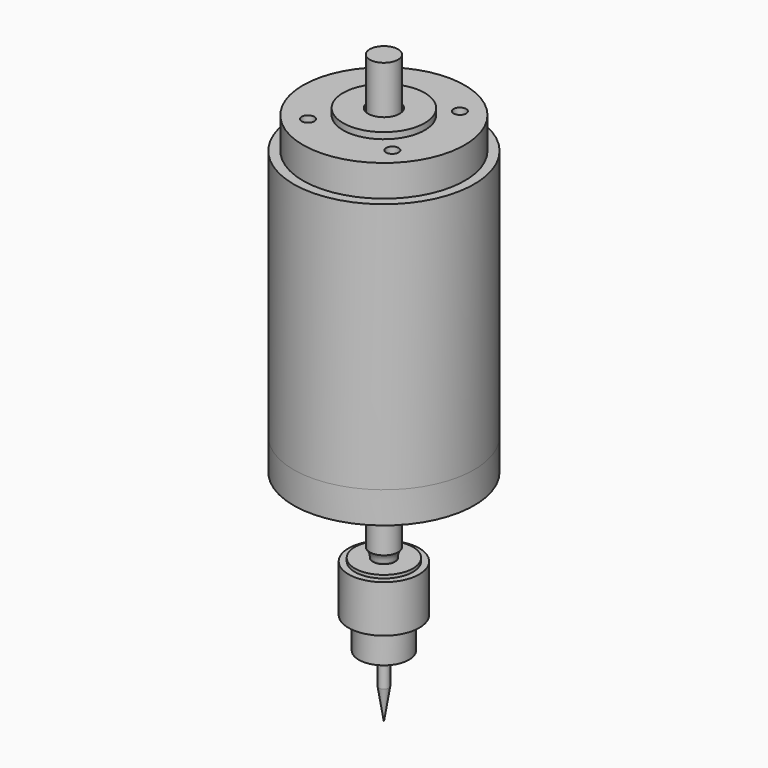
from build123d import *

# Parameters (mm, degrees)
F0_W      = 3
F0_H      = 80
F4_OFFSET = 0.5
F6_R      = 2
F7_DEPTH  = 10


# Not quite as in the source:
# - a fillet or chamfer that OpenCascade refuses, or shapes differently, is made with other operations: its cross-section is extruded or revolved along the edge and cut away or added


with BuildPart() as f1:
    # F0 (on Front) → F1 (revolve)
    with BuildSketch(Plane.XZ):
        Polygon((0, 100), (0, 102), (-13, 102), (-13, 100), (-25.75, 100), (-25.75, 90), (-25.75, 10), (-28.75, 10), (-28.75, 0), (-25.75, 0), (0, 0), align=None)
    revolve(axis=Axis((0, 0, 33.5), (0, 0, 1)))


with BuildPart() as f2:
    # F0 (on Front) → F2 (revolve)
    with BuildSketch(Plane.XZ):
        Polygon((4.5, 117), (0, 117), (0, 102), (0, 100), (0, 0), (0, -50), (1.5875, -50), (8, -50), (8, -41), (11.25, -40), (11.25, -25), (9.25, -25), (9.25, -24), (3.5, -24), (3.5, -21), (4.5, -21), align=None)
        Polygon((1.5875, -50), (0, -50), (0, -70), (1.5875, -60), align=None)
    revolve(axis=Axis((0, 0, 33.5), (0, 0, 1)))


with BuildPart() as f3:
    # F0 (on Front) → F3 (revolve)
    with BuildSketch(Plane.XZ):
        with Locations((-27.25, 50)):
            Rectangle(F0_W, F0_H)
    revolve(axis=Axis((0, 0, 33.5), (0, 0, 1)))


with BuildPart() as f1_1:
    add(f1.part)

    # F4: cut F2, made larger all round first
    f4_tool = offset(f2.part, amount=F4_OFFSET, kind=Kind.INTERSECTION, mode=Mode.PRIVATE)
    add(f4_tool, mode=Mode.SUBTRACT)

    # F6 (on face) → F7 (cut)
    with BuildSketch(Plane.XY.offset(100)):
        with Locations((-13.4350288425, 13.4350288425)):
            Circle(F6_R)
        with Locations((13.4350288425, 13.4350288425)):
            Circle(F6_R)
        with Locations((13.4350288425, -13.4350288425)):
            Circle(F6_R)
        with Locations((-13.4350288425, -13.4350288425)):
            Circle(F6_R)
    extrude(amount=-F7_DEPTH, mode=Mode.SUBTRACT)


with BuildPart() as f2_1:
    add(f2.part)

    # F5: fillet of radius 4 on 1 edges, made by hand

    # F5_s1 → F5_t2 (revolve)
    with BuildSketch(Plane.XZ):
        with BuildLine():
            ThreePointArc((3.5, -23.6457513111), (3.7583426132, -22.2315377487), (4.5, -21))
            Line((4.5, -21), (3.5, -21))
            Line((3.5, -21), (3.5, -23.6457513111))
        make_face()
    revolve(axis=Axis((0, 0, -21), (0, 0, 1)))


solid = Compound([f3.part, f1_1.part, f2_1.part])
